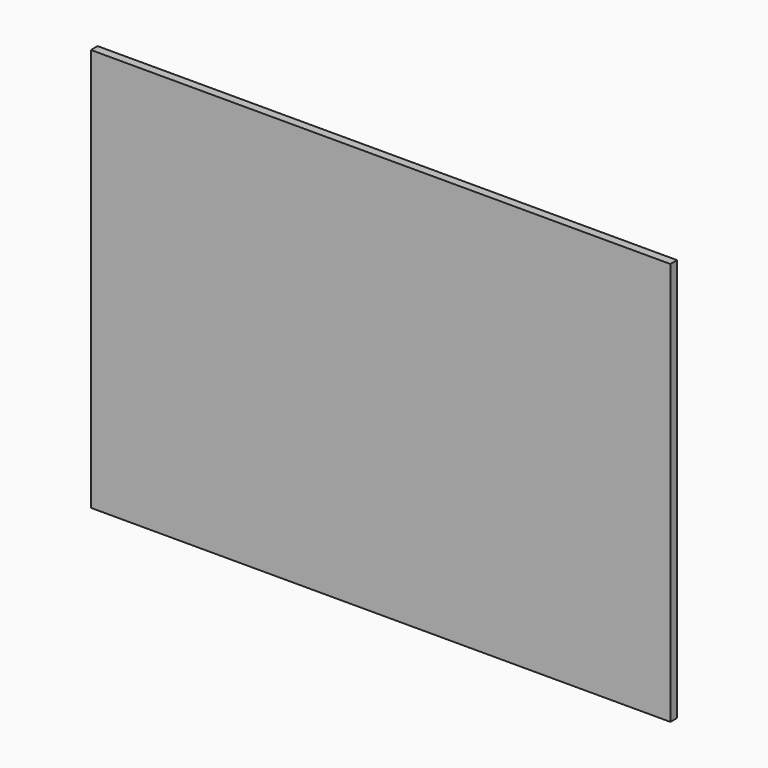
from build123d import *

# Parameters (mm, degrees)
F1_W     = 438.15
F1_H     = 304.8
F2_DEPTH = 6.35


# Not quite as in the source:
# - a variable given as a bare number and used for a length is read in inches; the dataset says mm whatever the document's units were


with BuildPart() as f2:
    # F1 (on Front) → F2 (new body)
    with BuildSketch(Plane.XZ):
        with Locations((219.075, -152.4)):
            Rectangle(F1_W, F1_H)
    extrude(amount=F2_DEPTH)


solid = f2.part
